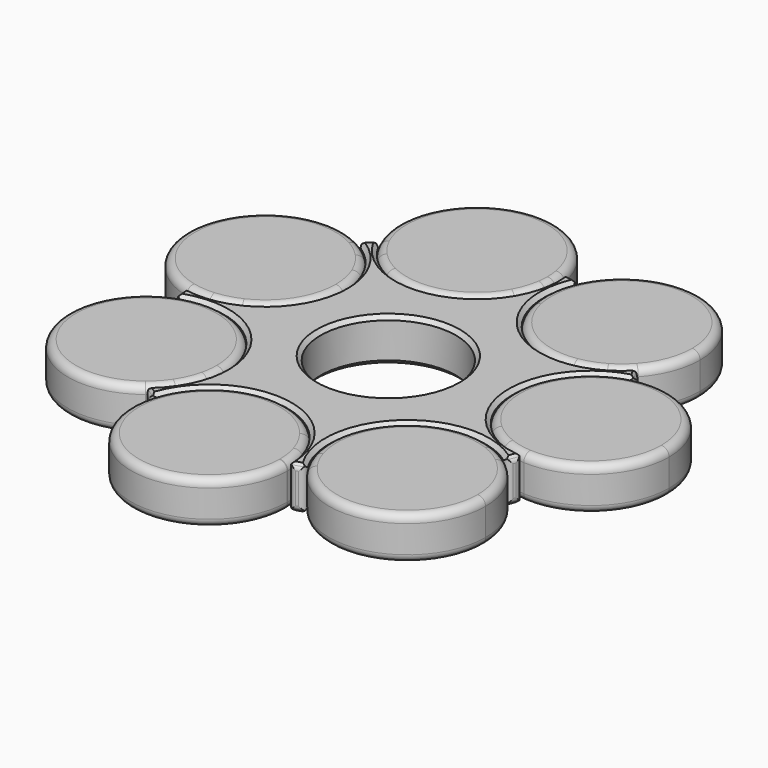
from build123d import *

# Parameters (mm, degrees)
F1_DEPTH     = 6.985
F0_R         = 15.875
F0_R_2       = 10.9855
F2_DEPTH     = 6.985
F3_T2_ANGLE  = 10.7784888428
F3_T4_ANGLE  = 179.0403967625
F3_T6_ANGLE  = 10.7784888428
F3_T8_ANGLE  = 179.0403967625
F3_T10_ANGLE = 10.7784888428
F3_T12_ANGLE = 179.0403967625
F3_T14_ANGLE = 10.7784888428
F3_T16_ANGLE = 179.0403967625
F3_T18_ANGLE = 10.7784888428
F3_T20_ANGLE = 179.0403967625
F3_T22_ANGLE = 10.7784888428
F3_T24_ANGLE = 179.0403967625
F3_T26_ANGLE = 10.7784888428
F3_T28_ANGLE = 179.0403967625
F3_T32_ANGLE = 10.7784888428
F3_T34_ANGLE = 179.0403967625
F3_T36_ANGLE = 10.7784888428
F3_T38_ANGLE = 179.0403967625
F3_T40_ANGLE = 10.7784888428
F3_T42_ANGLE = 179.0403967625
F3_T44_ANGLE = 10.7784888428
F3_T46_ANGLE = 179.0403967625
F3_T48_ANGLE = 10.7784888428
F3_T50_ANGLE = 179.0403967625
F3_T52_ANGLE = 10.7784888428
F3_T54_ANGLE = 179.0403967625
F3_T56_ANGLE = 10.7784888428
F3_T58_ANGLE = 179.0403967625
F4_T1_DEPTH  = 11.476520757
F4_T4_ANGLE  = 8.2156622332
F4_T6_ANGLE  = 8.2156622332
F4_T8_ANGLE  = 8.2156622332
F4_T10_ANGLE = 8.2156622332
F4_T12_ANGLE = 8.2156622332
F4_T14_ANGLE = 8.2156622332
F4_T16_ANGLE = 8.2156622332
F4_T18_ANGLE = 8.2156622332
F4_T20_ANGLE = 8.2156622332
F4_T22_ANGLE = 8.2156622332
F4_T24_ANGLE = 8.2156622332
F4_T26_ANGLE = 8.2156622332
F4_T28_ANGLE = 8.2156622332
F4_T30_ANGLE = 8.2156622332
F5_R         = 1.27
F5_2_R       = 1.27
F5_3_R       = 1.27
F5_4_R       = 1.27
F5_5_R       = 1.27
F5_6_R       = 1.27
F5_7_R       = 1.27


# Not quite as in the source:
# - a fillet or chamfer that OpenCascade refuses, or shapes differently, is made with other operations: its cross-section is extruded or revolved along the edge and cut away or added


with BuildPart() as f1:
    # F0 (on Top) → F1 (new body)
    with BuildSketch(Plane.XY):
        with BuildLine():
            ThreePointArc((-31.8336497569, -1.1619456784), (-29.7046840268, 11.5049172734), (-22.7461292131, 22.3012327108))
            ThreePointArc((-22.7461292131, 22.3012327108), (-40.7515737087, 15.7834866669), (-31.8336497569, -1.1619456784))
        make_face()
        with BuildLine():
            ThreePointArc((-17.1737559346, 16.0524405428), (-18.2331812497, 18.0756914999), (-19.6378436355, 19.8764829968))
            Line((-19.6378436355, 19.8764829968), (-28.9088086479, 11.1966668848))
            Line((-28.9088086479, 11.1966668848), (-27.9030072881, -1.4634422626))
            ThreePointArc((-27.9030072881, -1.4634422626), (-25.6518255474, -1.0785952746), (-23.5059707598, -0.2967809336))
            ThreePointArc((-23.5059707598, -0.2967809336), (-21.9210926211, 8.4902555072), (-17.1737559346, 16.0524405428))
        make_face()
        with BuildLine():
            ThreePointArc((-16.2088086479, 11.1966668848), (-16.4523812014, 13.6720285293), (-17.1737559346, 16.0524405428))
            ThreePointArc((-17.1737559346, 16.0524405428), (-21.9210926211, 8.4902555072), (-23.5059707598, -0.2967809336))
            ThreePointArc((-23.5059707598, -0.2967809336), (-18.1871940032, 4.3895397808), (-16.2088086479, 11.1966668848))
        make_face()
        with BuildLine():
            Line((-28.9088086479, 11.1966668848), (-19.6378436355, 19.8764829968))
            ThreePointArc((-19.6378436355, 19.8764829968), (-21.0973300411, 21.2101978293), (-22.7461292131, 22.3012327108))
            ThreePointArc((-22.7461292131, 22.3012327108), (-29.7046840268, 11.5049172734), (-31.8336497569, -1.1619456784))
            ThreePointArc((-31.8336497569, -1.1619456784), (-29.8800982223, -1.4661367764), (-27.9030072881, -1.4634422626))
            Line((-27.9030072881, -1.4634422626), (-28.9088086479, 11.1966668848))
        make_face()
    extrude(amount=F1_DEPTH)

    # F5
    f5_edges = [f1.edges().sort_by_distance(p)[0] for p in [
        (-25.983968, 23.555279, 6.985),
        (-25.983968, 23.555279, 0),
    ]]
    fillet(f5_edges, radius=F5_R)


with BuildPart() as f1b:
    # F0 (on Top) → F1, piece 2 (new body)
    with BuildSketch(Plane.XY):
        with BuildLine():
            ThreePointArc((-14.8877657288, 18.1926680805), (-5.4727175753, 17.4639424179), (1.8426417019, 23.4355160353))
            ThreePointArc((1.8426417019, 23.4355160353), (-7.0296286451, 22.4321880652), (-14.8877657288, 18.1926680805))
        make_face()
        with BuildLine():
            ThreePointArc((-20.7564016916, 24.164088301), (-9.5256610306, 30.3972557401), (3.253826235, 31.6882310872))
            ThreePointArc((3.253826235, 31.6882310872), (-13.0681638378, 41.7017062602), (-20.7564016916, 24.164088301))
        make_face()
        with BuildLine():
            Line((-9.2704407066, 29.582824339), (3.2960649305, 27.7462688473))
            ThreePointArc((3.2960649305, 27.7462688473), (3.3961417368, 28.6621239509), (3.4295592934, 29.582824339))
            ThreePointArc((3.4295592934, 29.582824339), (3.3855497754, 30.6391883486), (3.253826235, 31.6882310872))
            ThreePointArc((3.253826235, 31.6882310872), (-9.5256610306, 30.3972557401), (-20.7564016916, 24.164088301))
            ThreePointArc((-20.7564016916, 24.164088301), (-19.7762084095, 22.4470801612), (-18.541405719, 20.903008227))
            Line((-18.541405719, 20.903008227), (-9.2704407066, 29.582824339))
        make_face()
        with BuildLine():
            ThreePointArc((1.8426417019, 23.4355160353), (2.7639421174, 25.5252844383), (3.2960649305, 27.7462688473))
            Line((3.2960649305, 27.7462688473), (-9.2704407066, 29.582824339))
            Line((-9.2704407066, 29.582824339), (-18.541405719, 20.903008227))
            ThreePointArc((-18.541405719, 20.903008227), (-16.8369313704, 19.3829116417), (-14.8877657288, 18.1926680805))
            ThreePointArc((-14.8877657288, 18.1926680805), (-7.0296286451, 22.4321880652), (1.8426417019, 23.4355160353))
        make_face()
    extrude(amount=F1_DEPTH)

    # F5#2
    f5_2_edges = [f1b.edges().sort_by_distance(p)[0] for p in [
        (-20.383523, 35.730133, 6.985),
        (-20.383523, 35.730133, 0),
    ]]
    fillet(f5_2_edges, radius=F5_2_R)


with BuildPart() as f1c:
    # F0 (on Top) → F1, piece 3 (new body)
    with BuildSketch(Plane.XY):
        with BuildLine():
            ThreePointArc((4.941230551, 22.9826669671), (10.2416763937, 15.1673328929), (19.4714925539, 13.1711699558))
            ThreePointArc((19.4714925539, 13.1711699558), (13.1552890789, 19.4822254768), (4.941230551, 22.9826669671))
        make_face()
        with BuildLine():
            ThreePointArc((5.9508402008, 31.2940709321), (17.8263790097, 26.3998406435), (26.8035841622, 17.2133451328))
            ThreePointArc((26.8035841622, 17.2133451328), (29.2097507524, 21.1530342996), (30.0487581693, 25.6925116863))
            ThreePointArc((30.0487581693, 25.6925116863), (20.2242095948, 38.0627088998), (5.9508402008, 31.2940709321))
        make_face()
        with BuildLine():
            Line((4.7822525323, 27.529067178), (17.3487581693, 25.6925116863))
            Line((17.3487581693, 25.6925116863), (23.7479693763, 14.7225483351))
            ThreePointArc((23.7479693763, 14.722548335), (25.3730114714, 15.8486628992), (26.8035841622, 17.2133451328))
            ThreePointArc((26.8035841622, 17.2133451328), (17.8263790097, 26.3998406435), (5.9508402008, 31.2940709321))
            ThreePointArc((5.9508402008, 31.2940709321), (5.2195696967, 29.4571879004), (4.7822525323, 27.529067178))
        make_face()
        with BuildLine():
            Line((23.7479693763, 14.7225483351), (17.3487581693, 25.6925116863))
            Line((17.3487581693, 25.6925116863), (4.7822525323, 27.529067178))
            ThreePointArc((4.7822525323, 27.529067178), (4.6565155393, 25.2486907525), (4.941230551, 22.9826669671))
            ThreePointArc((4.941230551, 22.9826669671), (13.1552890789, 19.4822254768), (19.4714925539, 13.1711699558))
            ThreePointArc((19.4714925539, 13.1711699558), (21.6797606959, 13.7538175737), (23.7479693763, 14.722548335))
        make_face()
    extrude(amount=F1_DEPTH)

    # F5#3
    f5_3_edges = [f1c.edges().sort_by_distance(p)[0] for p in [
        (15.226024, 38.213853, 6.985),
        (15.226024, 38.213853, 0),
    ]]
    fillet(f5_3_edges, radius=F5_3_R)


with BuildPart() as f1d:
    # F0 (on Top) → F1, piece 4 (new body)
    with BuildSketch(Plane.XY):
        with BuildLine():
            ThreePointArc((-16.6806043295, -27.1383273951), (-6.3196834612, -43.2420028682), (8.2164667494, -30.776956457))
            ThreePointArc((8.2164667494, -30.776956457), (-4.6065509447, -31.5200105171), (-16.6806043295, -27.1383273951))
        make_face()
        with BuildLine():
            ThreePointArc((8.2168720305, -30.6754972311), (8.0707519168, -28.754533983), (7.6357539516, -26.8777740999))
            Line((7.6357539516, -26.8777740999), (-4.4831279695, -30.6754972311))
            Line((-4.4831279695, -30.6754972311), (-15.008306763, -23.5684154555))
            ThreePointArc((-15.008306763, -23.5684154555), (-15.9838163019, -25.2880889599), (-16.6806043295, -27.1383273951))
            ThreePointArc((-16.6806043295, -27.1383273951), (-4.6065509447, -31.5200105171), (8.2164667494, -30.776956457))
            ThreePointArc((8.2164667494, -30.776956457), (8.2167707098, -30.7262272488), (8.2168720305, -30.6754972311))
        make_face()
        with BuildLine():
            ThreePointArc((-11.8284521337, -20.3151780795), (-3.3994850722, -23.2607446468), (5.519910583, -22.8505870261))
            ThreePointArc((5.519910583, -22.8505870261), (-2.6465724778, -18.1089915941), (-11.8284521337, -20.3151780795))
        make_face()
        with BuildLine():
            ThreePointArc((7.6357539516, -26.8777740999), (6.7596208177, -24.7686706967), (5.519910583, -22.8505870261))
            ThreePointArc((5.519910583, -22.8505870261), (-3.3994850722, -23.2607446468), (-11.8284521337, -20.3151780795))
            ThreePointArc((-11.8284521337, -20.3151780795), (-13.5652316546, -21.7982570826), (-15.008306763, -23.5684154555))
            Line((-15.008306763, -23.5684154555), (-4.4831279695, -30.6754972311))
            Line((-4.4831279695, -30.6754972311), (7.6357539516, -26.8777740999))
        make_face()
    extrude(amount=F1_DEPTH)

    # F5#4
    f5_4_edges = [f1d.edges().sort_by_distance(p)[0] for p in [
        (-16.60201, -34.47322, 6.985),
        (-16.60201, -34.47322, 0),
    ]]
    fillet(f5_4_edges, radius=F5_4_R)


with BuildPart() as f1e:
    # F0 (on Top) → F1, piece 5 (new body)
    with BuildSketch(Plane.XY):
        with BuildLine():
            ThreePointArc((-14.0782540451, -15.6208091041), (-16.6294198765, -7.9859440091), (-23.2579650716, -3.4184500886))
            ThreePointArc((-23.2579650716, -3.4184500886), (-20.3055267446, -11.8450126174), (-14.4237003742, -18.5627478514))
            ThreePointArc((-14.4237003742, -18.5627478514), (-14.164911276, -17.1018844532), (-14.0782540451, -15.6208091041))
        make_face()
        with BuildLine():
            ThreePointArc((-14.4237003742, -18.5627478514), (-20.3055267446, -11.8450126174), (-23.2579650716, -3.4184500886))
            ThreePointArc((-23.2579650716, -3.4184500886), (-25.5003472466, -2.9852658148), (-27.7840554049, -2.9606999566))
            Line((-27.7840554049, -2.9606999566), (-26.7782540451, -15.6208091041))
            Line((-26.7782540451, -15.6208091041), (-16.2530752516, -22.7278908797))
            ThreePointArc((-16.2530752516, -22.7278908797), (-15.1503718853, -20.7278979498), (-14.4237003742, -18.5627478514))
        make_face()
        with BuildLine():
            ThreePointArc((-27.7840554049, -2.9606999566), (-29.7367705394, -3.2702147802), (-31.6177854273, -3.879048759))
            ThreePointArc((-31.6177854273, -3.879048759), (-27.5154740857, -16.0508585577), (-18.9395102671, -25.6130108626))
            ThreePointArc((-18.9395102671, -25.6130108626), (-17.4836646307, -24.2753228176), (-16.2530752516, -22.7278908797))
            Line((-16.2530752516, -22.7278908797), (-26.7782540451, -15.6208091041))
            Line((-26.7782540451, -15.6208091041), (-27.7840554049, -2.9606999566))
        make_face()
        with BuildLine():
            ThreePointArc((-18.9395102671, -25.6130108626), (-27.5154740857, -16.0508585577), (-31.6177854273, -3.879048759))
            ThreePointArc((-31.6177854273, -3.879048759), (-37.7482173964, -22.020020311), (-18.9395102671, -25.6130108626))
        make_face()
    extrude(amount=F1_DEPTH)

    # F5#5
    f5_5_edges = [f1e.edges().sort_by_distance(p)[0] for p in [
        (-21.938723, -27.362569, 6.985),
        (-21.938723, -27.362569, 0),
    ]]
    fillet(f5_5_edges, radius=F5_5_R)


with BuildPart() as f1f:
    # F0 (on Top) → F1, piece 6 (new body)
    with BuildSketch(Plane.XY):
        with BuildLine():
            ThreePointArc((8.5081265174, -21.9141626225), (16.0664381965, -17.1606615245), (21.3069162855, -9.9314681031))
            ThreePointArc((21.3069162855, -9.9314681031), (12.5080687942, -13.3599452647), (8.5081265174, -21.9141626225))
        make_face()
        with BuildLine():
            Line((21.1878849062, -22.6309102771), (25.7747046883, -10.7881452162))
            ThreePointArc((25.7747046883, -10.7881452162), (23.5794811738, -10.1581292202), (21.3069162855, -9.9314681031))
            ThreePointArc((21.3069162855, -9.9314681031), (16.0664381965, -17.1606615245), (8.5081265174, -21.9141626225))
            ThreePointArc((8.5081265174, -21.9141626225), (8.5847800537, -24.1967161638), (9.0690029851, -26.4286334083))
            Line((9.0690029851, -26.4286334083), (21.1878849062, -22.6309102771))
        make_face()
        with BuildLine():
            ThreePointArc((29.1852767182, -12.7652261038), (27.5571711747, -11.6435451502), (25.7747046883, -10.7881452162))
            Line((25.7747046883, -10.7881452162), (21.1878849062, -22.6309102771))
            Line((21.1878849062, -22.6309102771), (9.0690029851, -26.4286334083))
            ThreePointArc((9.0690029851, -26.4286334083), (9.8052776213, -28.2635163698), (10.8174120508, -29.9618919817))
            ThreePointArc((10.8174120508, -29.9618919817), (21.7711990142, -23.253951666), (29.1852767182, -12.7652261038))
        make_face()
        with BuildLine():
            ThreePointArc((33.8878849062, -22.6309102771), (32.6521091716, -17.1663369182), (29.1852767182, -12.7652261038))
            ThreePointArc((29.1852767182, -12.7652261038), (21.7711990142, -23.253951666), (10.8174120508, -29.9618919817))
            ThreePointArc((10.8174120508, -29.9618919817), (25.0339864868, -34.7345255482), (33.8878849062, -22.6309102771))
        make_face()
    extrude(amount=F1_DEPTH)

    # F5#6
    f5_6_edges = [f1f.edges().sort_by_distance(p)[0] for p in [
        (31.558358, -15.299929, 6.985),
        (31.558358, -15.299929, 0),
    ]]
    fillet(f5_6_edges, radius=F5_6_R)


with BuildPart() as f1g:
    # F0 (on Top) → F1, piece 7 (new body)
    with BuildSketch(Plane.XY):
        with BuildLine():
            ThreePointArc((23.5078442287, 0), (22.8849762218, 5.375556121), (21.0493794432, 10.4662488666))
            ThreePointArc((21.0493794432, 10.4662488666), (18.2438791461, 1.4494123423), (22.4379123667, -7.0113357433))
            ThreePointArc((22.4379123667, -7.0113357433), (23.238821926, -3.5462509462), (23.5078442287, 0))
        make_face()
        with BuildLine():
            Line((30.9039882935, 2.4552137021), (24.5047770865, 13.4251770534))
            ThreePointArc((24.5047770865, 13.4251770534), (22.6435112723, 12.1016907472), (21.0493794432, 10.4662488666))
            ThreePointArc((21.0493794432, 10.4662488666), (22.8849762218, 5.375556121), (23.5078442287, 0))
            ThreePointArc((23.5078442287, 0), (23.238821926, -3.5462509462), (22.4379123667, -7.0113357433))
            ThreePointArc((22.4379123667, -7.0113357433), (24.2702772839, -8.3745544506), (26.3171685115, -9.3875513588))
            Line((26.3171685115, -9.3875513588), (30.9039882935, 2.4552137021))
        make_face()
        with BuildLine():
            ThreePointArc((28.176978047, 14.8589798687), (26.2849053615, 14.2854323335), (24.5047770865, 13.4251770534))
            Line((24.5047770865, 13.4251770534), (30.9039882935, 2.4552137021))
            Line((30.9039882935, 2.4552137021), (26.3171685115, -9.3875513588))
            ThreePointArc((26.3171685115, -9.3875513588), (28.2107975045, -9.9559394826), (30.1696965218, -10.2235407949))
            ThreePointArc((30.1696965218, -10.2235407949), (31.4307372438, -5.1807461736), (31.8548485258, 0))
            ThreePointArc((31.8548485258, 0), (30.9217135861, 7.6536921482), (28.176978047, 14.8589798687))
        make_face()
        with BuildLine():
            ThreePointArc((43.6039882935, 2.4552137021), (38.8619079296, 12.3527646651), (28.176978047, 14.8589798687))
            ThreePointArc((28.176978047, 14.8589798687), (30.9217135861, 7.6536921482), (31.8548485258, 0))
            ThreePointArc((31.8548485258, 0), (31.4307372438, -5.1807461736), (30.1696965218, -10.2235407949))
            ThreePointArc((30.1696965218, -10.2235407949), (39.6207679311, -6.7810059115), (43.6039882935, 2.4552137021))
        make_face()
    extrude(amount=F1_DEPTH)

    # F5#7
    f5_7_edges = [f1g.edges().sort_by_distance(p)[0] for p in [
        (31.63828, 15.133968, 6.985),
        (31.63828, 15.133968, 0),
    ]]
    fillet(f5_7_edges, radius=F5_7_R)


with BuildPart() as f2:
    # F0 (on Top) → F2 (new body)
    with BuildSketch(Plane.XY):
        with BuildLine():
            ThreePointArc((21.0493794432, 10.4662488666), (20.3055267446, 11.8450126174), (19.4714925539, 13.1711699558))
            ThreePointArc((19.4714925539, 13.1711699558), (10.2416763937, 15.1673328929), (4.941230551, 22.9826669671))
            ThreePointArc((4.941230551, 22.9826669671), (3.3994850722, 23.2607446468), (1.8426417019, 23.4355160353))
            ThreePointArc((1.8426417019, 23.4355160353), (-5.4727175753, 17.4639424179), (-14.8877657288, 18.1926680805))
            ThreePointArc((-14.8877657288, 18.1926680805), (-16.0664381965, 17.1606615245), (-17.1737559346, 16.0524405428))
            ThreePointArc((-17.1737559346, 16.0524405428), (-16.4523812014, 13.6720285293), (-16.2088086479, 11.1966668848))
            ThreePointArc((-16.2088086479, 11.1966668848), (-18.1871940032, 4.3895397808), (-23.5059707598, -0.2967809336))
            ThreePointArc((-23.5059707598, -0.2967809336), (-23.4340058076, -1.8617497394), (-23.2579650716, -3.4184500886))
            ThreePointArc((-23.2579650716, -3.4184500886), (-16.6294198765, -7.9859440091), (-14.0782540451, -15.6208091041))
            ThreePointArc((-14.0782540451, -15.6208091041), (-14.164911276, -17.1018844532), (-14.4237003742, -18.5627478514))
            ThreePointArc((-14.4237003742, -18.5627478514), (-13.1552890789, -19.4822254768), (-11.8284521337, -20.3151780795))
            ThreePointArc((-11.8284521337, -20.3151780795), (-2.6465724778, -18.1089915941), (5.519910583, -22.8505870261))
            ThreePointArc((5.519910583, -22.8505870261), (7.0296286451, -22.4321880652), (8.5081265174, -21.9141626225))
            ThreePointArc((8.5081265174, -21.9141626225), (12.5080687942, -13.3599452647), (21.3069162855, -9.9314681031))
            ThreePointArc((21.3069162855, -9.9314681031), (21.9210926211, -8.4902555072), (22.4379123667, -7.0113357433))
            ThreePointArc((22.4379123667, -7.0113357433), (18.2438791461, 1.4494123423), (21.0493794432, 10.4662488666))
        make_face()
        Circle(F0_R, mode=Mode.SUBTRACT)
        Circle(F0_R)
        Circle(F0_R_2, mode=Mode.SUBTRACT)
        with BuildLine():
            ThreePointArc((-14.8877657288, 18.1926680805), (-16.8369313704, 19.3829116417), (-18.541405719, 20.903008227))
            Line((-18.541405719, 20.903008227), (-19.6378436355, 19.8764829968))
            ThreePointArc((-19.6378436355, 19.8764829968), (-18.2331812497, 18.0756914999), (-17.1737559346, 16.0524405428))
            ThreePointArc((-17.1737559346, 16.0524405428), (-16.0664381965, 17.1606615245), (-14.8877657288, 18.1926680805))
        make_face()
        with BuildLine():
            Line((-19.6378436355, 19.8764829968), (-18.541405719, 20.903008227))
            ThreePointArc((-18.541405719, 20.903008227), (-19.7762084095, 22.4470801612), (-20.7564016916, 24.164088301))
            ThreePointArc((-20.7564016916, 24.164088301), (-21.7711990142, 23.253951666), (-22.7461292131, 22.3012327108))
            ThreePointArc((-22.7461292131, 22.3012327108), (-21.0973300411, 21.2101978293), (-19.6378436355, 19.8764829968))
        make_face()
        with BuildLine():
            ThreePointArc((-23.2579650716, -3.4184500886), (-23.4340058076, -1.8617497394), (-23.5059707598, -0.2967809336))
            ThreePointArc((-23.5059707598, -0.2967809336), (-25.6518255474, -1.0785952746), (-27.9030072881, -1.4634422626))
            Line((-27.9030072881, -1.4634422626), (-27.7840554049, -2.9606999566))
            ThreePointArc((-27.7840554049, -2.9606999566), (-25.5003472466, -2.9852658148), (-23.2579650716, -3.4184500886))
        make_face()
        with BuildLine():
            ThreePointArc((-27.9030072881, -1.4634422626), (-29.8800982223, -1.4661367764), (-31.8336497569, -1.1619456784))
            ThreePointArc((-31.8336497569, -1.1619456784), (-31.7547920639, -2.5228070837), (-31.6177854273, -3.879048759))
            ThreePointArc((-31.6177854273, -3.879048759), (-29.7367705394, -3.2702147802), (-27.7840554049, -2.9606999566))
            Line((-27.7840554049, -2.9606999566), (-27.9030072881, -1.4634422626))
        make_face()
        with BuildLine():
            ThreePointArc((-15.008306763, -23.5684154555), (-13.5652316546, -21.7982570826), (-11.8284521337, -20.3151780795))
            ThreePointArc((-11.8284521337, -20.3151780795), (-13.1552890789, -19.4822254768), (-14.4237003742, -18.5627478514))
            ThreePointArc((-14.4237003742, -18.5627478514), (-15.1503718853, -20.7278979498), (-16.2530752516, -22.7278908797))
            Line((-16.2530752516, -22.7278908797), (-15.008306763, -23.5684154555))
        make_face()
        with BuildLine():
            ThreePointArc((-16.2530752516, -22.7278908797), (-17.4836646307, -24.2753228176), (-18.9395102671, -25.6130108626))
            ThreePointArc((-18.9395102671, -25.6130108626), (-17.8263790097, -26.3998406435), (-16.6806043295, -27.1383273951))
            ThreePointArc((-16.6806043295, -27.1383273951), (-15.9838163019, -25.2880889599), (-15.008306763, -23.5684154555))
            Line((-15.008306763, -23.5684154555), (-16.2530752516, -22.7278908797))
        make_face()
        with BuildLine():
            ThreePointArc((9.0690029851, -26.4286334083), (8.5847800537, -24.1967161638), (8.5081265174, -21.9141626225))
            ThreePointArc((8.5081265174, -21.9141626225), (7.0296286451, -22.4321880652), (5.519910583, -22.8505870261))
            ThreePointArc((5.519910583, -22.8505870261), (6.7596208177, -24.7686706967), (7.6357539516, -26.8777740999))
            Line((7.6357539516, -26.8777740999), (9.0690029851, -26.4286334083))
        make_face()
        with BuildLine():
            ThreePointArc((10.8174120508, -29.9618919817), (9.8052776213, -28.2635163698), (9.0690029851, -26.4286334083))
            Line((9.0690029851, -26.4286334083), (7.6357539516, -26.8777740999))
            ThreePointArc((7.6357539516, -26.8777740999), (8.0707519168, -28.754533983), (8.2168720305, -30.6754972311))
            ThreePointArc((8.2168720305, -30.6754972311), (8.2167707098, -30.7262272488), (8.2164667494, -30.776956457))
            ThreePointArc((8.2164667494, -30.776956457), (9.5256610306, -30.3972557401), (10.8174120508, -29.9618919817))
        make_face()
        with BuildLine():
            Line((25.7747046883, -10.7881452162), (26.3171685115, -9.3875513588))
            ThreePointArc((26.3171685115, -9.3875513588), (24.2702772839, -8.3745544506), (22.4379123667, -7.0113357433))
            ThreePointArc((22.4379123667, -7.0113357433), (21.9210926211, -8.4902555072), (21.3069162855, -9.9314681031))
            ThreePointArc((21.3069162855, -9.9314681031), (23.5794811738, -10.1581292202), (25.7747046883, -10.7881452162))
        make_face()
        with BuildLine():
            ThreePointArc((30.1696965218, -10.2235407949), (28.2107975045, -9.9559394826), (26.3171685115, -9.3875513588))
            Line((26.3171685115, -9.3875513588), (25.7747046883, -10.7881452162))
            ThreePointArc((25.7747046883, -10.7881452162), (27.5571711747, -11.6435451502), (29.1852767182, -12.7652261038))
            ThreePointArc((29.1852767182, -12.7652261038), (29.7046840268, -11.5049172734), (30.1696965218, -10.2235407949))
        make_face()
        with BuildLine():
            ThreePointArc((4.941230551, 22.9826669671), (4.6565155393, 25.2486907525), (4.7822525323, 27.529067178))
            Line((4.7822525323, 27.529067178), (3.2960649305, 27.7462688473))
            ThreePointArc((3.2960649305, 27.7462688473), (2.7639421174, 25.5252844383), (1.8426417019, 23.4355160353))
            ThreePointArc((1.8426417019, 23.4355160353), (3.3994850722, 23.2607446468), (4.941230551, 22.9826669671))
        make_face()
        with BuildLine():
            Line((3.2960649305, 27.7462688473), (4.7822525323, 27.529067178))
            ThreePointArc((4.7822525323, 27.529067178), (5.2195696967, 29.4571879004), (5.9508402008, 31.2940709321))
            ThreePointArc((5.9508402008, 31.2940709321), (4.6065509447, 31.5200105171), (3.253826235, 31.6882310872))
            ThreePointArc((3.253826235, 31.6882310872), (3.3855497754, 30.6391883486), (3.4295592934, 29.582824339))
            ThreePointArc((3.4295592934, 29.582824339), (3.3961417368, 28.6621239509), (3.2960649305, 27.7462688473))
        make_face()
        with BuildLine():
            ThreePointArc((26.8035841622, 17.2133451328), (25.3730114714, 15.8486628992), (23.7479693763, 14.722548335))
            Line((23.7479693763, 14.7225483351), (24.5047770865, 13.4251770534))
            ThreePointArc((24.5047770865, 13.4251770534), (26.2849053615, 14.2854323335), (28.176978047, 14.8589798687))
            ThreePointArc((28.176978047, 14.8589798687), (27.5154740857, 16.0508585577), (26.8035841622, 17.2133451328))
        make_face()
        with BuildLine():
            Line((24.5047770865, 13.4251770534), (23.7479693763, 14.7225483351))
            ThreePointArc((23.7479693763, 14.722548335), (21.6797606959, 13.7538175737), (19.4714925539, 13.1711699558))
            ThreePointArc((19.4714925539, 13.1711699558), (20.3055267446, 11.8450126174), (21.0493794432, 10.4662488666))
            ThreePointArc((21.0493794432, 10.4662488666), (22.6435112723, 12.1016907472), (24.5047770865, 13.4251770534))
        make_face()
    extrude(amount=F2_DEPTH)

    # F3: chamfer of 0.635 on 30 edges, made by hand

    # F3_s1 → F3_t2 (revolve, cut)
    with BuildSketch(Plane(origin=(0, 0, 0), x_dir=(0, 0, 1), z_dir=(0.9715326702, -0.2369056155, 0))):
        Polygon((6.35, -31.8548485258), (6.985, -31.2198485258), (6.985, -31.8548485258), align=None)
    revolve(axis=Axis((0, 0, 6.985), (0, 0, 1)), revolution_arc=F3_T2_ANGLE, mode=Mode.SUBTRACT)

    # F3_s3 → F3_t4 (revolve, cut)
    with BuildSketch(Plane(origin=(-9.0220721437, 29.6583780019, 0), x_dir=(0, 0, 1), z_dir=(-0.2910319852, 0.9567133236, 0))):
        Polygon((6.35, 12.4403939542), (6.985, 13.0753939542), (6.985, 12.4403939542), align=None)
    revolve(axis=Axis((-9.2704407066, 29.582824339, 6.985), (0, 0, -1)), revolution_arc=F3_T4_ANGLE, mode=Mode.SUBTRACT)

    # F3_s5 → F3_t6 (revolve, cut)
    with BuildSketch(Plane(origin=(0, 0, 0), x_dir=(0, 0, 1), z_dir=(0.7909609806, 0.6118665926, 0))):
        Polygon((6.35, -31.8548485258), (6.985, -31.2198485258), (6.985, -31.8548485258), align=None)
    revolve(axis=Axis((0, 0, 6.985), (0, 0, 1)), revolution_arc=F3_T6_ANGLE, mode=Mode.SUBTRACT)

    # F3_s7 → F3_t8 (revolve, cut)
    with BuildSketch(Plane(origin=(-28.813023614, 11.4379561848, 0), x_dir=(0, 0, 1), z_dir=(-0.9294440709, 0.3689630322, 0))):
        Polygon((6.35, 12.4403939542), (6.985, 13.0753939542), (6.985, 12.4403939542), align=None)
    revolve(axis=Axis((-28.9088086479, 11.1966668848, 6.985), (0, 0, -1)), revolution_arc=F3_T8_ANGLE, mode=Mode.SUBTRACT)

    # F3_s9 → F3_t10 (revolve, cut)
    with BuildSketch(Plane(origin=(0, 0, 0), x_dir=(0, 0, 1), z_dir=(0.0147795399, 0.9998907766, 0))):
        Polygon((6.35, -31.8548485258), (6.985, -31.2198485258), (6.985, -31.8548485258), align=None)
    revolve(axis=Axis((0, 0, 6.985), (0, 0, 1)), revolution_arc=F3_T10_ANGLE, mode=Mode.SUBTRACT)

    # F3_s11 → F3_t12 (revolve, cut)
    with BuildSketch(Plane(origin=(-26.9071806245, -15.3954799312, 0), x_dir=(0, 0, 1), z_dir=(-0.867965814, -0.496623948, 0))):
        Polygon((6.35, 12.4403939542), (6.985, 13.0753939542), (6.985, 12.4403939542), align=None)
    revolve(axis=Axis((-26.7782540451, -15.6208091041, 6.985), (0, 0, -1)), revolution_arc=F3_T12_ANGLE, mode=Mode.SUBTRACT)

    # F3_s13 → F3_t14 (revolve, cut)
    with BuildSketch(Plane(origin=(0, 0, 0), x_dir=(0, 0, 1), z_dir=(-0.7725311958, 0.6349768118, 0))):
        Polygon((6.35, -31.8548485258), (6.985, -31.2198485258), (6.985, -31.8548485258), align=None)
    revolve(axis=Axis((0, 0, 6.985), (0, 0, 1)), revolution_arc=F3_T14_ANGLE, mode=Mode.SUBTRACT)

    # F3_s15 → F3_t16 (revolve, cut)
    with BuildSketch(Plane(origin=(-4.7396818182, -30.6358056485, 0), x_dir=(0, 0, 1), z_dir=(-0.1528915959, -0.988242966, 0))):
        Polygon((6.35, 12.4403939542), (6.985, 13.0753939542), (6.985, 12.4403939542), align=None)
    revolve(axis=Axis((-4.4831279695, -30.6754972311, 6.985), (0, 0, -1)), revolution_arc=F3_T16_ANGLE, mode=Mode.SUBTRACT)

    # F3_s17 → F3_t18 (revolve, cut)
    with BuildSketch(Plane(origin=(0, 0, 0), x_dir=(0, 0, 1), z_dir=(-0.9781101843, -0.2080876435, 0))):
        Polygon((6.35, -31.8548485258), (6.985, -31.2198485258), (6.985, -31.8548485258), align=None)
    revolve(axis=Axis((0, 0, 6.985), (0, 0, 1)), revolution_arc=F3_T18_ANGLE, mode=Mode.SUBTRACT)

    # F3_s19 → F3_t20 (revolve, cut)
    with BuildSketch(Plane(origin=(20.9968940691, -22.8067448559, 0), x_dir=(0, 0, 1), z_dir=(0.6773131123, -0.7356948742, 0))):
        Polygon((6.35, 12.4403939542), (6.985, 13.0753939542), (6.985, 12.4403939542), align=None)
    revolve(axis=Axis((21.1878849062, -22.6309102771, 6.985), (0, 0, -1)), revolution_arc=F3_T20_ANGLE, mode=Mode.SUBTRACT)

    # F3_s21 → F3_t22 (revolve, cut)
    with BuildSketch(Plane(origin=(0, 0, 0), x_dir=(0, 0, 1), z_dir=(-0.4471522542, -0.894457859, 0))):
        Polygon((6.35, -31.8548485258), (6.985, -31.2198485258), (6.985, -31.8548485258), align=None)
    revolve(axis=Axis((0, 0, 6.985), (0, 0, 1)), revolution_arc=F3_T22_ANGLE, mode=Mode.SUBTRACT)

    # F3_s23 → F3_t24 (revolve, cut)
    with BuildSketch(Plane(origin=(30.9223804637, 2.196259986, 0), x_dir=(0, 0, 1), z_dir=(0.9974872323, 0.0708464634, 0))):
        Polygon((6.35, 12.4403939542), (6.985, 13.0753939542), (6.985, 12.4403939542), align=None)
    revolve(axis=Axis((30.9039882935, 2.4552137021, 6.985), (0, 0, -1)), revolution_arc=F3_T24_ANGLE, mode=Mode.SUBTRACT)

    # F3_s25 → F3_t26 (revolve, cut)
    with BuildSketch(Plane(origin=(0, 0, 0), x_dir=(0, 0, 1), z_dir=(0.4205204435, -0.9072830631, 0))):
        Polygon((6.35, -31.8548485258), (6.985, -31.2198485258), (6.985, -31.8548485258), align=None)
    revolve(axis=Axis((0, 0, 6.985), (0, 0, 1)), revolution_arc=F3_T26_ANGLE, mode=Mode.SUBTRACT)

    # F3_s27 → F3_t28 (revolve, cut)
    with BuildSketch(Plane(origin=(17.5626836676, 25.5454362629, 0), x_dir=(0, 0, 1), z_dir=(0.5665331213, 0.824038969, 0))):
        Polygon((6.35, 12.4403939542), (6.985, 13.0753939542), (6.985, 12.4403939542), align=None)
    revolve(axis=Axis((17.3487581693, 25.6925116863, 6.985), (0, 0, -1)), revolution_arc=F3_T28_ANGLE, mode=Mode.SUBTRACT)

    # F3_s29 → F3_t30 (revolve, cut)
    with BuildSketch(Plane.XZ):
        Polygon((10.9855, 6.35), (11.6205, 6.985), (10.9855, 6.985), align=None)
    revolve(axis=Axis((0, 0, 6.985), (0, 0, 1)), mode=Mode.SUBTRACT)

    # F3_s31 → F3_t32 (revolve, cut)
    with BuildSketch(Plane(origin=(0, 0, 0), x_dir=(0, 0, 1), z_dir=(0.9715326702, -0.2369056155, 0))):
        Polygon((0.635, -31.8548485258), (0, -31.2198485258), (0, -31.8548485258), align=None)
    revolve(axis=Axis((0, 0, 0), (0, 0, 1)), revolution_arc=F3_T32_ANGLE, mode=Mode.SUBTRACT)

    # F3_s33 → F3_t34 (revolve, cut)
    with BuildSketch(Plane(origin=(-9.0220721437, 29.6583780019, 0), x_dir=(0, 0, 1), z_dir=(-0.2910319852, 0.9567133236, 0))):
        Polygon((0.635, 12.4403939542), (0, 13.0753939542), (0, 12.4403939542), align=None)
    revolve(axis=Axis((-9.2704407066, 29.582824339, 0), (0, 0, -1)), revolution_arc=F3_T34_ANGLE, mode=Mode.SUBTRACT)

    # F3_s35 → F3_t36 (revolve, cut)
    with BuildSketch(Plane(origin=(0, 0, 0), x_dir=(0, 0, 1), z_dir=(0.7909609806, 0.6118665926, 0))):
        Polygon((0.635, -31.8548485258), (0, -31.2198485258), (0, -31.8548485258), align=None)
    revolve(axis=Axis((0, 0, 0), (0, 0, 1)), revolution_arc=F3_T36_ANGLE, mode=Mode.SUBTRACT)

    # F3_s37 → F3_t38 (revolve, cut)
    with BuildSketch(Plane(origin=(-28.813023614, 11.4379561848, 0), x_dir=(0, 0, 1), z_dir=(-0.9294440709, 0.3689630322, 0))):
        Polygon((0.635, 12.4403939542), (0, 13.0753939542), (0, 12.4403939542), align=None)
    revolve(axis=Axis((-28.9088086479, 11.1966668848, 0), (0, 0, -1)), revolution_arc=F3_T38_ANGLE, mode=Mode.SUBTRACT)

    # F3_s39 → F3_t40 (revolve, cut)
    with BuildSketch(Plane(origin=(0, 0, 0), x_dir=(0, 0, 1), z_dir=(0.0147795399, 0.9998907766, 0))):
        Polygon((0.635, -31.8548485258), (0, -31.2198485258), (0, -31.8548485258), align=None)
    revolve(axis=Axis((0, 0, 0), (0, 0, 1)), revolution_arc=F3_T40_ANGLE, mode=Mode.SUBTRACT)

    # F3_s41 → F3_t42 (revolve, cut)
    with BuildSketch(Plane(origin=(-26.9071806245, -15.3954799312, 0), x_dir=(0, 0, 1), z_dir=(-0.867965814, -0.496623948, 0))):
        Polygon((0.635, 12.4403939542), (0, 13.0753939542), (0, 12.4403939542), align=None)
    revolve(axis=Axis((-26.7782540451, -15.6208091041, 0), (0, 0, -1)), revolution_arc=F3_T42_ANGLE, mode=Mode.SUBTRACT)

    # F3_s43 → F3_t44 (revolve, cut)
    with BuildSketch(Plane(origin=(0, 0, 0), x_dir=(0, 0, 1), z_dir=(-0.7725311958, 0.6349768118, 0))):
        Polygon((0.635, -31.8548485258), (0, -31.2198485258), (0, -31.8548485258), align=None)
    revolve(axis=Axis((0, 0, 0), (0, 0, 1)), revolution_arc=F3_T44_ANGLE, mode=Mode.SUBTRACT)

    # F3_s45 → F3_t46 (revolve, cut)
    with BuildSketch(Plane(origin=(-4.7396818182, -30.6358056485, 0), x_dir=(0, 0, 1), z_dir=(-0.1528915959, -0.988242966, 0))):
        Polygon((0.635, 12.4403939542), (0, 13.0753939542), (0, 12.4403939542), align=None)
    revolve(axis=Axis((-4.4831279695, -30.6754972311, 0), (0, 0, -1)), revolution_arc=F3_T46_ANGLE, mode=Mode.SUBTRACT)

    # F3_s47 → F3_t48 (revolve, cut)
    with BuildSketch(Plane(origin=(0, 0, 0), x_dir=(0, 0, 1), z_dir=(-0.9781101843, -0.2080876435, 0))):
        Polygon((0.635, -31.8548485258), (0, -31.2198485258), (0, -31.8548485258), align=None)
    revolve(axis=Axis((0, 0, 0), (0, 0, 1)), revolution_arc=F3_T48_ANGLE, mode=Mode.SUBTRACT)

    # F3_s49 → F3_t50 (revolve, cut)
    with BuildSketch(Plane(origin=(20.9968940691, -22.8067448559, 0), x_dir=(0, 0, 1), z_dir=(0.6773131123, -0.7356948742, 0))):
        Polygon((0.635, 12.4403939542), (0, 13.0753939542), (0, 12.4403939542), align=None)
    revolve(axis=Axis((21.1878849062, -22.6309102771, 0), (0, 0, -1)), revolution_arc=F3_T50_ANGLE, mode=Mode.SUBTRACT)

    # F3_s51 → F3_t52 (revolve, cut)
    with BuildSketch(Plane(origin=(0, 0, 0), x_dir=(0, 0, 1), z_dir=(-0.4471522542, -0.894457859, 0))):
        Polygon((0.635, -31.8548485258), (0, -31.2198485258), (0, -31.8548485258), align=None)
    revolve(axis=Axis((0, 0, 0), (0, 0, 1)), revolution_arc=F3_T52_ANGLE, mode=Mode.SUBTRACT)

    # F3_s53 → F3_t54 (revolve, cut)
    with BuildSketch(Plane(origin=(30.9223804637, 2.196259986, 0), x_dir=(0, 0, 1), z_dir=(0.9974872323, 0.0708464634, 0))):
        Polygon((0.635, 12.4403939542), (0, 13.0753939542), (0, 12.4403939542), align=None)
    revolve(axis=Axis((30.9039882935, 2.4552137021, 0), (0, 0, -1)), revolution_arc=F3_T54_ANGLE, mode=Mode.SUBTRACT)

    # F3_s55 → F3_t56 (revolve, cut)
    with BuildSketch(Plane(origin=(0, 0, 0), x_dir=(0, 0, 1), z_dir=(0.4205204435, -0.9072830631, 0))):
        Polygon((0.635, -31.8548485258), (0, -31.2198485258), (0, -31.8548485258), align=None)
    revolve(axis=Axis((0, 0, 0), (0, 0, 1)), revolution_arc=F3_T56_ANGLE, mode=Mode.SUBTRACT)

    # F3_s57 → F3_t58 (revolve, cut)
    with BuildSketch(Plane(origin=(17.5626836676, 25.5454362629, 0), x_dir=(0, 0, 1), z_dir=(0.5665331213, 0.824038969, 0))):
        Polygon((0.635, 12.4403939542), (0, 13.0753939542), (0, 12.4403939542), align=None)
    revolve(axis=Axis((17.3487581693, 25.6925116863, 0), (0, 0, -1)), revolution_arc=F3_T58_ANGLE, mode=Mode.SUBTRACT)

    # F3_s59 → F3_t60 (revolve, cut)
    with BuildSketch(Plane.XZ):
        Polygon((10.9855, 0.635), (11.6205, 0), (10.9855, 0), align=None)
    revolve(axis=Axis((0, 0, 0), (0, 0, 1)), mode=Mode.SUBTRACT)

    # F4: fillet of radius 0.889 on 28 edges, made by hand

    # F4_s2 → F4_t1 (cut)
    with BuildSketch(Plane.XY.offset(-2.2457603785)):
        with BuildLine():
            ThreePointArc((-21.9246636033, 23.1093163137), (-22.1987354129, 22.3907094307), (-21.8097291735, 21.727244771))
            ThreePointArc((-21.8097291735, 21.727244771), (-22.271721344, 22.0243661843), (-22.7461292131, 22.3012327108))
            ThreePointArc((-22.7461292131, 22.3012327108), (-22.3390506174, 22.7089892358), (-21.9246636033, 23.1093163137))
        make_face()
        with BuildLine():
            ThreePointArc((-20.2452649656, 23.1919533121), (-20.8816986565, 23.6237673533), (-21.6167802989, 23.3975679102))
            ThreePointArc((-21.6167802989, 23.3975679102), (-21.1900572528, 23.7847187964), (-20.7564016916, 24.164088301))
            ThreePointArc((-20.7564016916, 24.164088301), (-20.5113472561, 23.6724927117), (-20.2452649656, 23.1919533121))
        make_face()
        with BuildLine():
            ThreePointArc((-31.7373951982, -2.732969198), (-31.3464466919, -3.3952912303), (-30.5851877102, -3.5048173547))
            ThreePointArc((-30.5851877102, -3.5048173547), (-31.1055339921, -3.6807652071), (-31.6177854273, -3.879048759))
            ThreePointArc((-31.6177854273, -3.879048759), (-31.6827729628, -3.3065498621), (-31.7373951982, -2.732969198))
        make_face()
        with BuildLine():
            ThreePointArc((-30.7549154813, -1.3684391458), (-31.4893312091, -1.5967913908), (-31.7707972707, -2.312534407))
            ThreePointArc((-31.7707972707, -2.312534407), (-31.8074265546, -1.7375242659), (-31.8336497569, -1.1619456784))
            ThreePointArc((-31.8336497569, -1.1619456784), (-31.296515907, -1.2768592423), (-30.7549154813, -1.3684391458))
        make_face()
        with BuildLine():
            ThreePointArc((-17.651220884, -26.5172731612), (-16.8896442609, -26.6245683437), (-16.329376077, -26.0976805271))
            ThreePointArc((-16.329376077, -26.0976805271), (-16.5162451069, -26.6142053237), (-16.6806043295, -27.1383273951))
            ThreePointArc((-16.6806043295, -27.1383273951), (-17.1687210564, -26.8321894725), (-17.651220884, -26.5172731612))
        make_face()
        with BuildLine():
            ThreePointArc((-18.1054873536, -24.8983690158), (-18.384855096, -25.614933649), (-18.0007558916, -26.2812511486))
            ThreePointArc((-18.0007558916, -26.2812511486), (-18.4731549075, -25.951376117), (-18.9395102671, -25.6130108626))
            ThreePointArc((-18.9395102671, -25.6130108626), (-18.5147697474, -25.2647101437), (-18.1054873536, -24.8983690158))
        make_face()
        with BuildLine():
            ThreePointArc((4.3977868665, 31.5498152971), (3.6650764036, 31.3160492032), (3.3889002683, 30.5982484291))
            ThreePointArc((3.3889002683, 30.5982484291), (3.3331517365, 31.1447006238), (3.253826235, 31.6882310872))
            ThreePointArc((3.253826235, 31.6882310872), (3.8264324764, 31.6241962602), (4.3977868665, 31.5498152971))
        make_face()
        with BuildLine():
            ThreePointArc((4.81511314, 31.4888243676), (5.4502788935, 31.0551474433), (5.5094829973, 30.2883318963))
            ThreePointArc((5.5094829973, 30.2883318963), (5.7192842339, 30.7959748229), (5.9508402008, 31.2940709321))
            ThreePointArc((5.9508402008, 31.2940709321), (5.3838573588, 31.3965834852), (4.81511314, 31.4888243676))
        make_face()
        with BuildLine():
            ThreePointArc((26.0356186871, 16.4281469296), (26.7690109343, 16.6597651947), (27.4086141273, 16.2326598628))
            ThreePointArc((27.4086141273, 16.2326598628), (27.1105338706, 16.7257384846), (26.8035841622, 17.2133451328))
            ThreePointArc((26.8035841622, 17.2133451328), (26.4280935755, 16.8124402574), (26.0356186871, 16.4281469296))
        make_face()
        with BuildLine():
            ThreePointArc((27.621128174, 15.8683538212), (27.6780852713, 15.101368099), (27.1154778903, 14.5769787932))
            ThreePointArc((27.1154778903, 14.5769787932), (27.6431780436, 14.7294597691), (28.176978047, 14.8589798687))
            ThreePointArc((28.176978047, 14.8589798687), (27.9036175685, 15.366180436), (27.621128174, 15.8683538212))
        make_face()
        with BuildLine():
            ThreePointArc((29.0769852047, -10.112684281), (29.7153342431, -10.5416618027), (29.7801959164, -11.3080195341))
            ThreePointArc((29.7801959164, -11.3080195341), (29.979850306, -10.7675415128), (30.1696965218, -10.2235407949))
            ThreePointArc((30.1696965218, -10.2235407949), (29.6221419172, -10.179930534), (29.0769852047, -10.112684281))
        make_face()
        with BuildLine():
            ThreePointArc((29.6278703247, -11.7013108079), (29.0637289097, -12.2240494357), (28.302964877, -12.1111366573))
            ThreePointArc((28.302964877, -12.1111366573), (28.7511949684, -12.4286389171), (29.1852767182, -12.7652261038))
            ThreePointArc((29.1852767182, -12.7652261038), (29.4113846191, -12.2352698944), (29.6278703247, -11.7013108079))
        make_face()
        with BuildLine():
            ThreePointArc((10.2227888008, -29.0384579669), (10.2854047845, -29.805002452), (9.7266827751, -30.3335295802))
            ThreePointArc((9.7266827751, -30.3335295802), (10.2737279836, -30.1526431333), (10.8174120508, -29.9618919817))
            ThreePointArc((10.8174120508, -29.9618919817), (10.5101132138, -29.5066060006), (10.2227888008, -29.0384579669))
        make_face()
        with BuildLine():
            ThreePointArc((9.3242218225, -30.4596497355), (8.5637918871, -30.3445084201), (8.177742036, -29.6793191828))
            ThreePointArc((8.177742036, -29.6793191828), (8.2089756645, -30.2277190007), (8.2164667494, -30.776956457))
            ThreePointArc((8.2164667494, -30.776956457), (8.7717791686, -30.6233124403), (9.3242218225, -30.4596497355))
        make_face()
    extrude(amount=F4_T1_DEPTH, mode=Mode.SUBTRACT)

    # F4_s3 → F4_t4 (revolve, cut)
    with BuildSketch(Plane(origin=(0, 0, 0), x_dir=(0, 0, 1), z_dir=(0.7770799914, 0.6294018486, 0))):
        with BuildLine():
            ThreePointArc((1.0032358569, -31.8548485258), (0.6630302856, -31.7871774302), (0.3746179285, -31.5944664543))
            Line((0.3746179285, -31.5944664543), (0.635, -31.8548485258))
            Line((0.635, -31.8548485258), (1.0032358569, -31.8548485258))
        make_face()
    revolve(axis=Axis((0, 0, 0.635), (0, 0, 1)), revolution_arc=F4_T4_ANGLE, mode=Mode.SUBTRACT)

    # F4_s5 → F4_t6 (revolve, cut)
    with BuildSketch(Plane(origin=(0, 0, 0), x_dir=(0, 0, 1), z_dir=(0.7770799914, 0.6294018486, 0))):
        with BuildLine():
            ThreePointArc((5.9817641431, -31.8548485258), (6.3219697144, -31.7871774302), (6.6103820715, -31.5944664543))
            Line((6.6103820715, -31.5944664543), (6.35, -31.8548485258))
            Line((6.35, -31.8548485258), (5.9817641431, -31.8548485258))
        make_face()
    revolve(axis=Axis((0, 0, 6.35), (0, 0, 1)), revolution_arc=F4_T6_ANGLE, mode=Mode.SUBTRACT)

    # F4_s7 → F4_t8 (revolve, cut)
    with BuildSketch(Plane(origin=(0, 0, 0), x_dir=(0, 0, 1), z_dir=(-0.0075847305, 0.9999712355, 0))):
        with BuildLine():
            ThreePointArc((0.3746179285, -31.5944664543), (0.6630302856, -31.7871774302), (1.0032358569, -31.8548485258))
            Line((1.0032358569, -31.8548485258), (0.635, -31.8548485258))
            Line((0.635, -31.8548485258), (0.3746179285, -31.5944664543))
        make_face()
    revolve(axis=Axis((0, 0, 0.635), (0, 0, 1)), revolution_arc=F4_T8_ANGLE, mode=Mode.SUBTRACT)

    # F4_s9 → F4_t10 (revolve, cut)
    with BuildSketch(Plane(origin=(0, 0, 0), x_dir=(0, 0, 1), z_dir=(-0.0075847305, 0.9999712355, 0))):
        with BuildLine():
            ThreePointArc((6.6103820715, -31.5944664543), (6.3219697144, -31.7871774302), (5.9817641431, -31.8548485258))
            Line((5.9817641431, -31.8548485258), (6.35, -31.8548485258))
            Line((6.35, -31.8548485258), (6.6103820715, -31.5944664543))
        make_face()
    revolve(axis=Axis((0, 0, 6.35), (0, 0, 1)), revolution_arc=F4_T10_ANGLE, mode=Mode.SUBTRACT)

    # F4_s11 → F4_t12 (revolve, cut)
    with BuildSketch(Plane(origin=(0, 0, 0), x_dir=(0, 0, 1), z_dir=(-0.7865379956, 0.6175418864, 0))):
        with BuildLine():
            ThreePointArc((0.3746179285, -31.5944664543), (0.6630302856, -31.7871774302), (1.0032358569, -31.8548485258))
            Line((1.0032358569, -31.8548485258), (0.635, -31.8548485258))
            Line((0.635, -31.8548485258), (0.3746179285, -31.5944664543))
        make_face()
    revolve(axis=Axis((0, 0, 0.635), (0, 0, 1)), revolution_arc=F4_T12_ANGLE, mode=Mode.SUBTRACT)

    # F4_s13 → F4_t14 (revolve, cut)
    with BuildSketch(Plane(origin=(0, 0, 0), x_dir=(0, 0, 1), z_dir=(-0.7865379956, 0.6175418864, 0))):
        with BuildLine():
            ThreePointArc((6.6103820715, -31.5944664543), (6.3219697144, -31.7871774302), (5.9817641431, -31.8548485258))
            Line((5.9817641431, -31.8548485258), (6.35, -31.8548485258))
            Line((6.35, -31.8548485258), (6.6103820715, -31.5944664543))
        make_face()
    revolve(axis=Axis((0, 0, 6.35), (0, 0, 1)), revolution_arc=F4_T14_ANGLE, mode=Mode.SUBTRACT)

    # F4_s15 → F4_t16 (revolve, cut)
    with BuildSketch(Plane(origin=(0, 0, 0), x_dir=(0, 0, 1), z_dir=(0.9765876302, -0.2151199678, 0))):
        with BuildLine():
            ThreePointArc((1.0032358569, -31.8548485258), (0.6630302856, -31.7871774302), (0.3746179285, -31.5944664543))
            Line((0.3746179285, -31.5944664543), (0.635, -31.8548485258))
            Line((0.635, -31.8548485258), (1.0032358569, -31.8548485258))
        make_face()
    revolve(axis=Axis((0, 0, 0.635), (0, 0, 1)), revolution_arc=F4_T16_ANGLE, mode=Mode.SUBTRACT)

    # F4_s17 → F4_t18 (revolve, cut)
    with BuildSketch(Plane(origin=(0, 0, 0), x_dir=(0, 0, 1), z_dir=(0.9765876302, -0.2151199678, 0))):
        with BuildLine():
            ThreePointArc((5.9817641431, -31.8548485258), (6.3219697144, -31.7871774302), (6.6103820715, -31.5944664543))
            Line((6.6103820715, -31.5944664543), (6.35, -31.8548485258))
            Line((6.35, -31.8548485258), (5.9817641431, -31.8548485258))
        make_face()
    revolve(axis=Axis((0, 0, 6.35), (0, 0, 1)), revolution_arc=F4_T18_ANGLE, mode=Mode.SUBTRACT)

    # F4_s19 → F4_t20 (revolve, cut)
    with BuildSketch(Plane(origin=(0, 0, 0), x_dir=(0, 0, 1), z_dir=(0.4407048647, -0.8976520608, 0))):
        with BuildLine():
            ThreePointArc((1.0032358569, -31.8548485258), (0.6630302856, -31.7871774302), (0.3746179285, -31.5944664543))
            Line((0.3746179285, -31.5944664543), (0.635, -31.8548485258))
            Line((0.635, -31.8548485258), (1.0032358569, -31.8548485258))
        make_face()
    revolve(axis=Axis((0, 0, 0.635), (0, 0, 1)), revolution_arc=F4_T20_ANGLE, mode=Mode.SUBTRACT)

    # F4_s21 → F4_t22 (revolve, cut)
    with BuildSketch(Plane(origin=(0, 0, 0), x_dir=(0, 0, 1), z_dir=(0.4407048647, -0.8976520608, 0))):
        with BuildLine():
            ThreePointArc((5.9817641431, -31.8548485258), (6.3219697144, -31.7871774302), (6.6103820715, -31.5944664543))
            Line((6.6103820715, -31.5944664543), (6.35, -31.8548485258))
            Line((6.35, -31.8548485258), (5.9817641431, -31.8548485258))
        make_face()
    revolve(axis=Axis((0, 0, 6.35), (0, 0, 1)), revolution_arc=F4_T22_ANGLE, mode=Mode.SUBTRACT)

    # F4_s23 → F4_t24 (revolve, cut)
    with BuildSketch(Plane(origin=(0, 0, 0), x_dir=(0, 0, 1), z_dir=(-0.4270376526, -0.9042338432, 0))):
        with BuildLine():
            ThreePointArc((0.3746179285, -31.5944664543), (0.6630302856, -31.7871774302), (1.0032358569, -31.8548485258))
            Line((1.0032358569, -31.8548485258), (0.635, -31.8548485258))
            Line((0.635, -31.8548485258), (0.3746179285, -31.5944664543))
        make_face()
    revolve(axis=Axis((0, 0, 0.635), (0, 0, 1)), revolution_arc=F4_T24_ANGLE, mode=Mode.SUBTRACT)

    # F4_s25 → F4_t26 (revolve, cut)
    with BuildSketch(Plane(origin=(0, 0, 0), x_dir=(0, 0, 1), z_dir=(-0.4270376526, -0.9042338432, 0))):
        with BuildLine():
            ThreePointArc((6.6103820715, -31.5944664543), (6.3219697144, -31.7871774302), (5.9817641431, -31.8548485258))
            Line((5.9817641431, -31.8548485258), (6.35, -31.8548485258))
            Line((6.35, -31.8548485258), (6.6103820715, -31.5944664543))
        make_face()
    revolve(axis=Axis((0, 0, 6.35), (0, 0, 1)), revolution_arc=F4_T26_ANGLE, mode=Mode.SUBTRACT)

    # F4_s27 → F4_t28 (revolve, cut)
    with BuildSketch(Plane(origin=(0, 0, 0), x_dir=(0, 0, 1), z_dir=(-0.9732121076, -0.2299090987, 0))):
        with BuildLine():
            ThreePointArc((0.3746179285, -31.5944664543), (0.6630302856, -31.7871774302), (1.0032358569, -31.8548485258))
            Line((1.0032358569, -31.8548485258), (0.635, -31.8548485258))
            Line((0.635, -31.8548485258), (0.3746179285, -31.5944664543))
        make_face()
    revolve(axis=Axis((0, 0, 0.635), (0, 0, 1)), revolution_arc=F4_T28_ANGLE, mode=Mode.SUBTRACT)

    # F4_s29 → F4_t30 (revolve, cut)
    with BuildSketch(Plane(origin=(0, 0, 0), x_dir=(0, 0, 1), z_dir=(-0.9732121076, -0.2299090987, 0))):
        with BuildLine():
            ThreePointArc((6.6103820715, -31.5944664543), (6.3219697144, -31.7871774302), (5.9817641431, -31.8548485258))
            Line((5.9817641431, -31.8548485258), (6.35, -31.8548485258))
            Line((6.35, -31.8548485258), (6.6103820715, -31.5944664543))
        make_face()
    revolve(axis=Axis((0, 0, 6.35), (0, 0, 1)), revolution_arc=F4_T30_ANGLE, mode=Mode.SUBTRACT)


solid = Compound([f1.part, f1b.part, f1c.part, f1d.part, f1e.part, f1f.part, f1g.part, f2.part])
